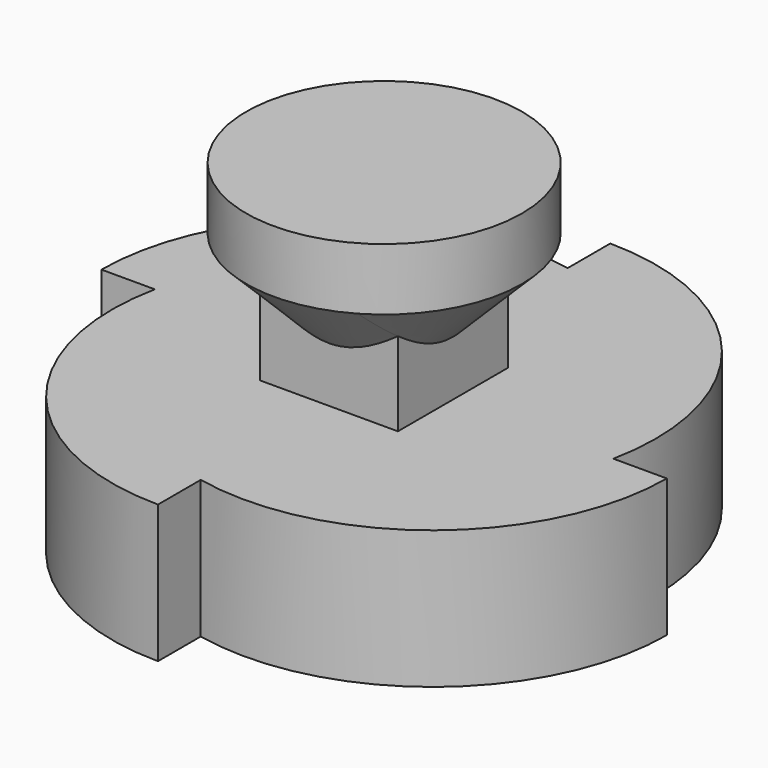
from build123d import *

# Parameters (mm, degrees)
F0_W     = 41
F0_H     = 41
F0_W_2   = 10
F0_H_2   = 10
F1_DEPTH = 10
F2_DEPTH = 25
F3_R     = 10
F4_DEPTH = 8
F6_DEPTH = 25
F7_DEPTH = 1.5
F8_DEPTH = 3


# Not quite as in the source:
# - a fillet or chamfer that OpenCascade refuses, or shapes differently, is made with other operations: its cross-section is extruded or revolved along the edge and cut away or added


with BuildPart() as f1:
    # F0 (on Top) → F1 (new body)
    with BuildSketch(Plane.XY):
        Rectangle(F0_W, F0_H)
        Rectangle(F0_W_2, F0_H_2, mode=Mode.SUBTRACT)
        Rectangle(F0_W_2, F0_H_2)
    extrude(amount=F1_DEPTH)

    # F0 (on Top) → F2 (join)
    with BuildSketch(Plane.XY):
        Rectangle(F0_W_2, F0_H_2)
    extrude(amount=F2_DEPTH)

    # F3 (on face) → F4 (join)
    with BuildSketch(Plane.XY.offset(25)):
        Circle(F3_R)
    extrude(amount=-F4_DEPTH)

    # F5 (on face) → F6 (cut)
    with BuildSketch(Plane(origin=(0, 0, 0), x_dir=(1, 0, 0), z_dir=(0, 0, -1))):
        with BuildLine():
            Line((0, 20.5), (0, 16.625))
            ThreePointArc((0, 16.625), (14.2014511666, 13.1849661001), (20.5, 0))
            Line((20.5, 0), (20.5, 20.5))
            Line((20.5, 20.5), (0, 20.5))
        make_face()
        with BuildLine():
            Line((20.5, -20.5), (20.5, 0))
            Line((20.5, 0), (16.625, 0))
            ThreePointArc((16.625, 0), (13.15340166, -14.1758531755), (0, -20.5))
            Line((0, -20.5), (20.5, -20.5))
        make_face()
        with BuildLine():
            ThreePointArc((0, -16.625), (-14.1919455674, -13.1732449101), (-20.5, 0))
            Line((-20.5, 0), (-20.5, -20.5))
            Line((-20.5, -20.5), (0, -20.5))
            Line((0, -20.5), (0, -16.625))
        make_face()
        with BuildLine():
            ThreePointArc((-16.625, 0), (-13.1636820987, 14.1841903605), (0, 20.5))
            Line((0, 20.5), (-20.5, 20.5))
            Line((-20.5, 20.5), (-20.5, 0))
            Line((-20.5, 0), (-16.625, 0))
        make_face()
    extrude(amount=-F6_DEPTH, mode=Mode.SUBTRACT)

    # F7 (cut): a face of the model
    f7_faces = [f1.faces().sort_by_distance(p)[0] for p in [
        (0, 0, 25),
    ]]
    extrude(f7_faces, amount=-F7_DEPTH, mode=Mode.SUBTRACT)

    # F8 (add): a face of the model
    f8_faces = [f1.faces().sort_by_distance(p)[0] for p in [
        (-9.7171572875, 0, 17),
    ]]
    extrude(f8_faces, amount=F8_DEPTH)

    # F9: chamfer of 5 on 1 edges, made by hand


with BuildPart() as f9_tool2:
    # F9_s3 → F9_t4 (revolve)
    with BuildSketch(Plane.XZ):
        Polygon((5, 14), (10, 19), (10, 14), align=None)
    revolve(axis=Axis((0, 0, 14), (0, 0, 1)))

    split(bisect_by=Plane.YZ.offset(5), keep=Keep.TOP)


with BuildPart() as f1_1:
    add(f1.part)

    # F9_t1: cut F9_tool2
    add(f9_tool2.part, mode=Mode.SUBTRACT)


with BuildPart() as f9_tool7:
    # F9_s8 → F9_t9 (revolve)
    with BuildSketch(Plane.XZ):
        Polygon((5, 14), (10, 19), (10, 14), align=None)
    revolve(axis=Axis((0, 0, 14), (0, 0, 1)))

    split(bisect_by=Plane.XZ.offset(-5), keep=Keep.BOTTOM)


with BuildPart() as f1_2:
    add(f1_1.part)

    # F9_t6: cut F9_tool7
    add(f9_tool7.part, mode=Mode.SUBTRACT)


with BuildPart() as f9_tool12:
    # F9_s13 → F9_t14 (revolve)
    with BuildSketch(Plane.XZ):
        Polygon((5, 14), (10, 19), (10, 14), align=None)
    revolve(axis=Axis((0, 0, 14), (0, 0, 1)))

    split(bisect_by=Plane.YZ.offset(-5), keep=Keep.BOTTOM)


with BuildPart() as f1_3:
    add(f1_2.part)

    # F9_t11: cut F9_tool12
    add(f9_tool12.part, mode=Mode.SUBTRACT)


with BuildPart() as f9_tool17:
    # F9_s18 → F9_t19 (revolve)
    with BuildSketch(Plane.XZ):
        Polygon((5, 14), (10, 19), (10, 14), align=None)
    revolve(axis=Axis((0, 0, 14), (0, 0, 1)))

    split(bisect_by=Plane.XZ.offset(5), keep=Keep.TOP)


with BuildPart() as f1_4:
    add(f1_3.part)

    # F9_t16: cut F9_tool17
    add(f9_tool17.part, mode=Mode.SUBTRACT)


solid = f1_4.part
